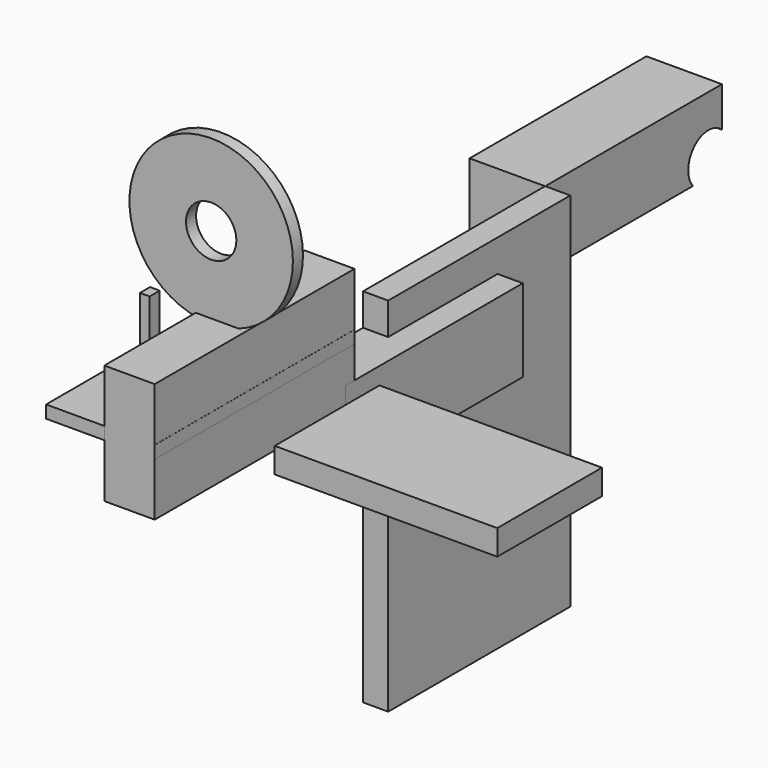
from build123d import *

# Parameters (mm, degrees)
F0_W      = 251.9057244062
F0_H      = 120.4088665545
F1_DEPTH  = 50.8
F2_W      = 9.7853951156
F2_H      = 118.5759752989
F3_DEPTH  = 12.7
F5_DEPTH  = 12.7
F6_W      = 109.9998280406
F6_H      = 251.6520246863
F7_DEPTH  = 12.7
F9_D      = 50.8
F10_W     = 224.532097578
F10_H     = 132.0753507316
F11_DEPTH = 25.4
F12_W     = 229.6327352524
F12_H     = 365.1259541512
F13_DEPTH = 25.4
F18_W     = 223.8502129912
F18_H     = 83.3336301148
F19_DEPTH = 50.8
F20_W     = 222.9283154011
F20_H     = 75.5738317966
F21_DEPTH = 76.2
F23_D     = 50.8
F25_D     = 50.8


# Not quite as in the source:
# - the program builds the solid bodies; features that only make, move or delete a surface that nothing else refers to are left out


with BuildPart() as f1:
    # F0 (on Right) → F1 (new body)
    with BuildSketch(Plane.YZ):
        with Locations((-1.9939765334, 6.465299055)):
            Rectangle(F0_W, F0_H)
    extrude(amount=F1_DEPTH)


with BuildPart() as f3:
    # F2 (on Front) → F3 (new body)
    with BuildSketch(Plane.XZ):
        with Locations((-51.3733271509, 6.7634359002)):
            Rectangle(F2_W, F2_H)
    extrude(amount=F3_DEPTH)


with BuildPart() as f5:
    # F4 (on Front) → F5 (new body)
    with BuildSketch(Plane.XZ):
        with BuildLine():
            ThreePointArc((39.5767722748, 65.4155793169), (81.8127708761, 95.209089617), (98.0136903376, 144.2912966013))
            ThreePointArc((98.0136903376, 144.2912966013), (-50.6854651748, 193.3735035856), (39.5767722748, 65.4155793169))
        make_face()
    extrude(amount=F5_DEPTH)

    # F9 (through all)
    with Locations(Plane(origin=(0, 0, 0), x_dir=(-1, 0, 0), z_dir=(0, 1, 0))):
        with Locations((-15.5636528507, 144.2912966013)):
            Hole(F9_D / 2)


with BuildPart() as f7:
    # F6 (on Top) → F7 (new body)
    with BuildSketch(Plane.XY):
        with Locations((-4.1358657181, -1.6805864871)):
            Rectangle(F6_W, F6_H)
    extrude(amount=F7_DEPTH)


with BuildPart() as f11:
    # F10 (on Top) → F11 (new body)
    with BuildSketch(Plane.XY):
        with Locations((253.1674355268, -23.22778292)):
            Rectangle(F10_W, F10_H)
    extrude(amount=F11_DEPTH)


with BuildPart() as f13:
    # F12 (on Right) → F13 (new body)
    with BuildSketch(Plane.YZ):
        with Locations((313.0736649036, -182.5629770756)):
            Rectangle(F12_W, F12_H)
    extrude(amount=F13_DEPTH)

    # F23 (through all)
    with Locations(Plane.YZ.offset(25.4)):
        with Locations((322.5499093533, -236.1082434654)):
            Hole(F23_D / 2)


with BuildPart() as f19:
    # F18 (on Right) → F19 (new body)
    with BuildSketch(Plane.YZ):
        with Locations((224.2599911988, -74.0652363747)):
            Rectangle(F18_W, F18_H)
    extrude(amount=F19_DEPTH)


with BuildPart() as f21:
    # F20 (on face) → F21 (new body)
    with BuildSketch(Plane(origin=(0, 0, 0), x_dir=(0, -1, 0), z_dir=(-1, 0, 0))):
        with Locations((-539.3541902304, -37.8398001194)):
            Rectangle(F20_W, F20_H)
    extrude(amount=F21_DEPTH)

    # F25 (through all)
    with Locations(Plane.YZ):
        with Locations((633.7370872498, -59.328019619)):
            Hole(F25_D / 2)


solid = Compound([f1.part, f3.part, f5.part, f7.part, f11.part, f13.part, f19.part, f21.part])
